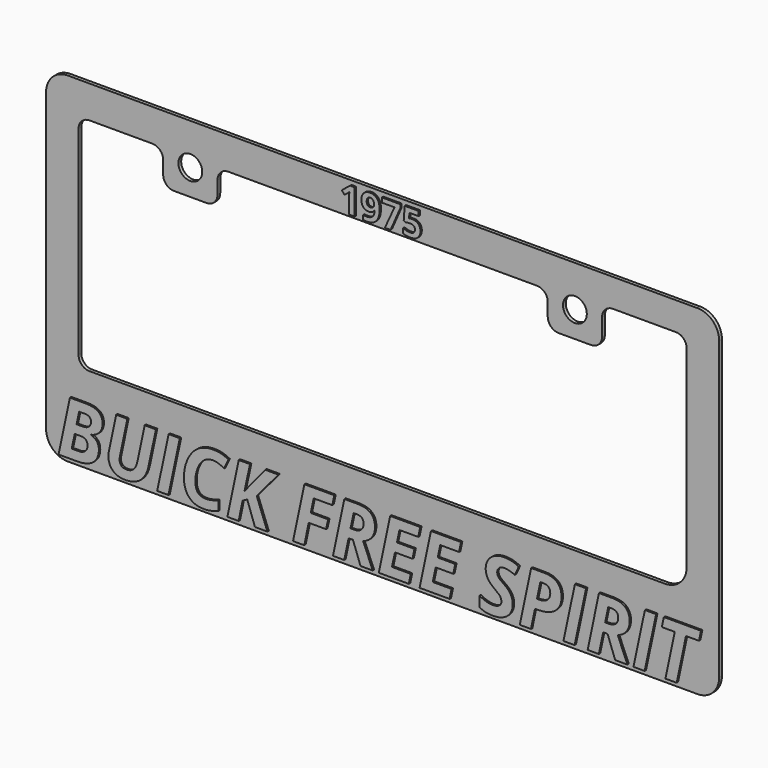
from build123d import *

# Parameters (mm, degrees)
F1_DEPTH      = 1.6
F2_W          = 25.1
F2_H          = 16
F3_DEPTH      = 1.6
F4_R          = 5
F5_W          = 39.1
F5_H          = 7
F6_DEPTH      = 25
F7_R          = 5
F8_R          = 5.5
F9_DEPTH      = 25
F10_TEXT_SIZE = 16.6666666667
F11_DEPTH     = 0.8
F12_TEXT_SIZE = 34.7618271685
F13_DEPTH     = 0.8


# Not quite as in the source:
# - Text() gives the source's letters only with a copy of the font that has no kerning and outlines rounded to 1/6400 em; it was checked with that copy


with BuildPart() as f1:
    # F0 (on Front) → F1 (new body)
    with BuildSketch(Plane.XZ):
        with BuildLine():
            ThreePointArc((155.5, 68.5), (152.5710678119, 75.5710678119), (145.5, 78.5))
            Line((145.5, 78.5), (-145.5, 78.5))
            ThreePointArc((-145.5, 78.5), (-152.5710678119, 75.5710678119), (-155.5, 68.5))
            Line((-155.5, 68.5), (-155.5, -68.5))
            ThreePointArc((-155.5, -68.5), (-152.5710678119, -75.5710678119), (-145.5, -78.5))
            Line((-145.5, -78.5), (145.5, -78.5))
            ThreePointArc((145.5, -78.5), (152.5710678119, -75.5710678119), (155.5, -68.5))
            Line((155.5, -68.5), (155.5, 68.5))
        make_face()
        with BuildLine():
            Line((-135.5, 63.5), (135.5, 63.5))
            ThreePointArc((135.5, 63.5), (139.0355339059, 62.0355339059), (140.5, 58.5))
            Line((140.5, 58.5), (140.5, -28.5))
            ThreePointArc((140.5, -28.5), (137.5710678119, -35.5710678119), (130.5, -38.5))
            Line((130.5, -38.5), (-135.5, -38.5))
            ThreePointArc((-135.5, -38.5), (-139.0355339059, -37.0355339059), (-140.5, -33.5))
            Line((-140.5, -33.5), (-140.5, 58.5))
            ThreePointArc((-140.5, 58.5), (-139.0355339059, 62.0355339059), (-135.5, 63.5))
        make_face(mode=Mode.SUBTRACT)
    extrude(amount=F1_DEPTH)

    # F2 (on face) → F3 (join, through all)
    with BuildSketch(Plane.XZ.offset(1.6)):
        with Locations((-88.85, 55.5)):
            Rectangle(F2_W, F2_H)
        with Locations((88.85, 55.5)):
            Rectangle(F2_W, F2_H)
    extrude(amount=-F3_DEPTH)

    # F4
    f4_edges = [f1.edges().sort_by_distance(p)[0] for p in [
        (-101.4, -0.8, 47.5),
        (-101.4, -0.8, 63.5),
        (-76.3, -0.8, 47.5),
        (-76.3, -0.8, 63.5),
        (101.4, -0.8, 47.5),
        (101.4, -0.8, 63.5),
        (76.3, -0.8, 47.5),
        (76.3, -0.8, 63.5),
    ]]
    fillet(f4_edges, radius=F4_R)

    # F5 (on face) → F6 (cut)
    with BuildSketch(Plane.XZ.offset(1.6)):
        with Locations((120.95, 62)):
            Rectangle(F5_W, F5_H)
    extrude(amount=-F6_DEPTH, mode=Mode.SUBTRACT)

    # F7
    f7_edges = [f1.edges().sort_by_distance(p)[0] for p in [
        (101.4, -0.8, 65.5),
        (140.5, -0.8, 65.5),
    ]]
    fillet(f7_edges, radius=F7_R)

    # F8 (on face) → F9 (cut)
    with BuildSketch(Plane.XZ.offset(1.6)):
        with Locations((-88.85, 59.5)):
            Circle(F8_R)
        with Locations((88.85, 59.5)):
            Circle(F8_R)
    extrude(amount=-F9_DEPTH, mode=Mode.SUBTRACT)

    # F10 (on face) → F11 (join)
    with BuildSketch(Plane.XZ.offset(1.6)):
        with Locations((-19.1927083333, 64.75)):
            Text('1975', F10_TEXT_SIZE, font='Open Sans', font_style=FontStyle.BOLD, text_align=(TextAlign.LEFT, TextAlign.BOTTOM))
    extrude(amount=F11_DEPTH)

    # F12 (on face) → F13 (join)
    with BuildSketch(Plane.XZ.offset(1.6)):
        with Locations((-150, -76.5)):
            Text('BUICK FREE SPIRIT', F12_TEXT_SIZE, font='Open Sans', font_style=FontStyle.BOLDITALIC, text_align=(TextAlign.LEFT, TextAlign.BOTTOM))
    extrude(amount=F13_DEPTH)


solid = f1.part
